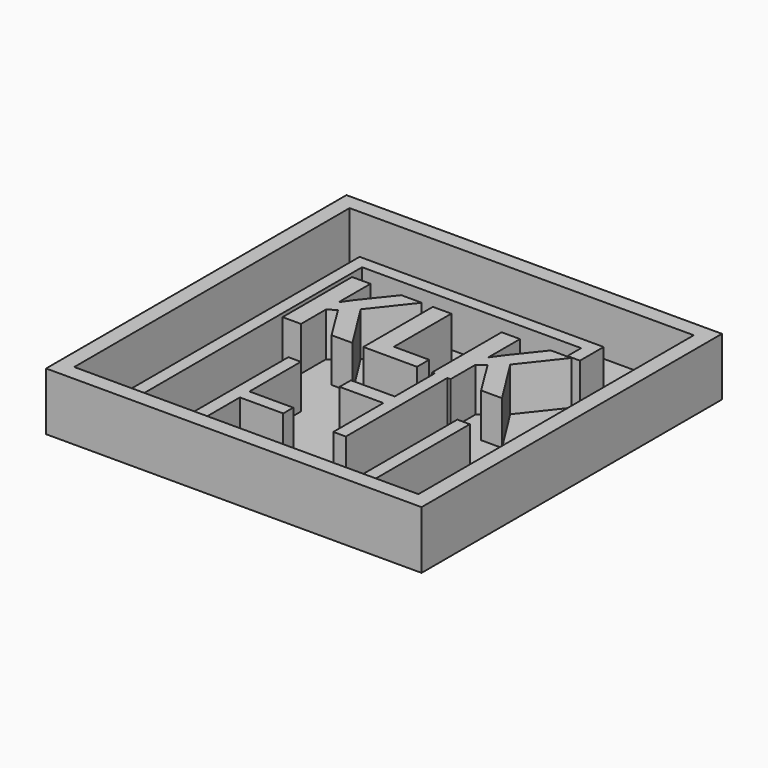
from build123d import *

# Parameters (mm, degrees)
F0_W         = 38.1
F0_H         = 38.1
F1_DEPTH     = 0.79375
F2_W         = 38.1
F2_H         = 38.1
F2_W_2       = 34.925
F2_H_2       = 34.925
F3_DEPTH     = 5.08
F4_TEXT_SIZE = 12.3472222222
F5_DEPTH     = 4.445
F4_R         = 1.27
F6_DEPTH     = 0.396875


# Not quite as in the source:
# - Text() gives the source's letters only with a copy of the font that has no kerning and outlines rounded to 1/6400 em; it was checked with that copy


with BuildPart() as f1:
    # F0 (on Top) → F1 (new body)
    with BuildSketch(Plane.XY):
        with Locations((3.1849592924, 1.5763216418)):
            Rectangle(F0_W, F0_H)
    extrude(amount=F1_DEPTH)

    # F2 (on face) → F3 (join)
    with BuildSketch(Plane.XY.offset(0.79375)):
        with Locations((3.1849592924, 1.5763216418)):
            Rectangle(F2_W, F2_H)
        with Locations((3.1849592924, 1.5763216418)):
            Rectangle(F2_W_2, F2_H_2, mode=Mode.SUBTRACT)
    extrude(amount=F3_DEPTH)

    # F4 (on face) → F5 (join)
    with BuildSketch(Plane.XY.offset(0.79375)):
        Polygon((5.8324856489, -3.01509563), (3.5024592924, -3.01509563), (3.5024592924, -4.4561783582), (5.8324856489, -4.4561783582), (7.1024856489, -4.4561783582), (7.9474592924, -4.4561783582), (7.9474592924, -10.8061783582), (9.2174592924, -10.8061783582), (9.2174592924, -4.3531266924), (9.2174592924, 2.06490437), (7.9474592924, 2.06490437), (7.9474592924, -3.01509563), (7.1024856489, -3.01509563), align=None)
        with Locations((-8.608015968, 2.06490437)):
            Text('KLK', F4_TEXT_SIZE, font='Open Sans', font_style=FontStyle.BOLD, text_align=(TextAlign.LEFT, TextAlign.BOTTOM))
        Polygon((-2.8475407076, -10.8061783582), (-2.8475407076, -15.8861783582), (-1.5350215835, -15.8861783582), (-1.5350215835, -10.8061783582), (2.8674592924, -10.8061783582), (2.8674592924, -9.5361783582), (-1.5775407076, -9.5361783582), (-1.5775407076, -3.01509563), (-2.8475407076, -3.01509563), (-2.8475407076, -9.5361783582), align=None)
        Polygon((14.2974592924, -3.01509563), (14.2974592924, -15.8861783582), (15.5674592924, -15.8861783582), (15.5674592924, -10.8061783582), (15.5674592924, -3.01509563), align=None)
        Polygon((-9.1975407076, 13.9588216418), (-9.1975407076, -15.8861783582), (-7.9275407076, -15.8861783582), (-7.9275407076, 8.7163262069), (-7.9275407076, 10.5404062197), (-7.9275407076, 12.6888216418), (14.2974592924, 12.6888216418), (14.2974592924, 10.95490437), (15.5674592924, 10.95490437), (15.5674592924, 12.6888216418), (15.5674592924, 13.9588216418), (-7.9275407076, 13.9588216418), align=None)
    extrude(amount=F5_DEPTH)

    # F4 (on face) → F6 (cut)
    with BuildSketch(Plane.XY.offset(0.79375)):
        with Locations((-11.7375407076, -12.6743260771)):
            Circle(F4_R)
        with Locations((-5.3875407076, -12.6743260771)):
            Circle(F4_R)
    extrude(amount=-F6_DEPTH, mode=Mode.SUBTRACT)


solid = f1.part
